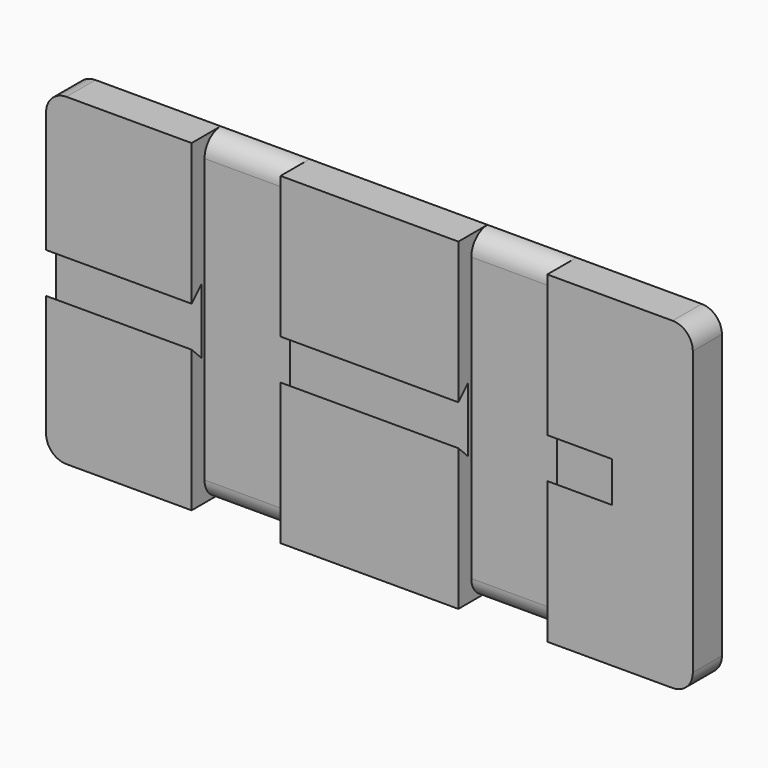
from build123d import *

# Parameters (mm, degrees)
F0_W     = 18
F0_H     = 40
F0_W_2   = 11
F0_W_3   = 22
F1_DEPTH = 4.5
F2_W     = 11
F2_H     = 40
F3_DEPTH = 2
F5_DEPTH = 70
F6_R     = 2.49999


# Not quite as in the source:
# - a fillet or chamfer is up to 0.001 mm smaller than in the source, because OpenCascade refuses the exact size


with BuildPart() as f1:
    # F0 (on Front) → F1 (new body)
    with BuildSketch(Plane.XZ):
        with Locations((-31, 0)):
            Rectangle(F0_W, F0_H)
        with Locations((-16.5, 0)):
            Rectangle(F0_W_2, F0_H)
        Rectangle(F0_W_3, F0_H)
        with Locations((16.5, 0)):
            Rectangle(F0_W_2, F0_H)
        with Locations((31, 0)):
            Rectangle(F0_W, F0_H)
    extrude(amount=-F1_DEPTH)

    # F2 (on Front) → F3 (cut)
    with BuildSketch(Plane.XZ):
        with Locations((-16.5, 0)):
            Rectangle(F2_W, F2_H)
        with Locations((16.5, 0)):
            Rectangle(F2_W, F2_H)
    extrude(amount=-F3_DEPTH, mode=Mode.SUBTRACT)

    # F4 (on face) → F5 (cut)
    with BuildSketch(Plane(origin=(-40, 0, 0), x_dir=(0, -1, 0), z_dir=(-1, 0, 0))):
        Polygon((0, -2.5), (0, 0), (0, 2.5), (-1.5, 4), (-1.5, 0), (-1.5, -4), align=None)
    extrude(amount=-F5_DEPTH, mode=Mode.SUBTRACT)

    # F6 (radius 2.5 in the source; OpenCascade refuses exactly that, so slightly less here)
    f6_edges = [f1.edges().sort_by_distance(p)[0] for p in [
        (-16.5, 2, 20),
        (16.5, 2, 20),
        (16.5, 2, -20),
        (-16.5, 2, -20),
        (-40, 2.25, 20),
        (-40, 2.25, -20),
        (40, 2.25, -20),
        (40, 2.25, 20),
    ]]
    fillet(f6_edges, radius=F6_R)


solid = f1.part
